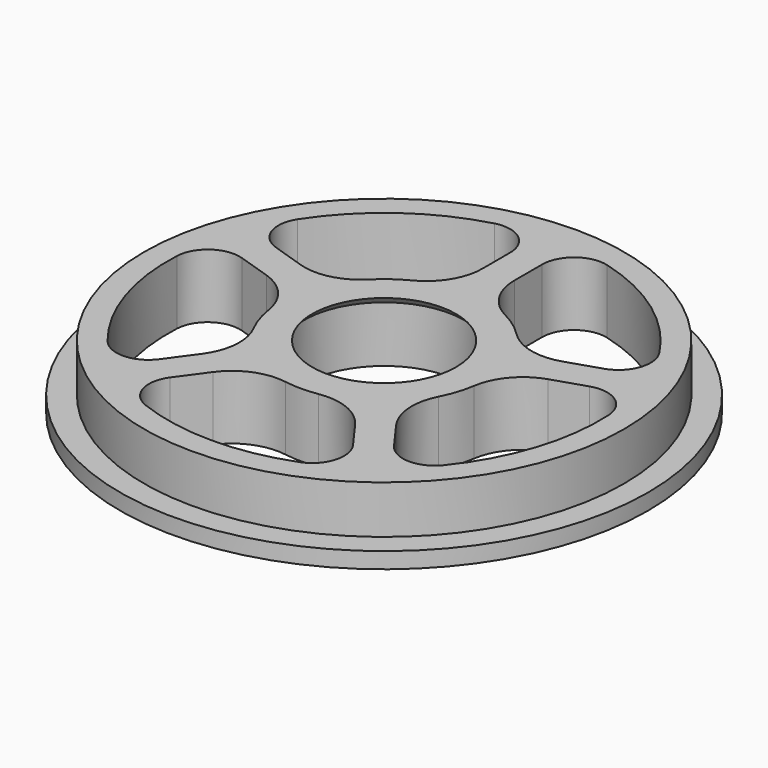
from build123d import *

# Parameters (mm, degrees)
F0_R     = 30
F0_R_2   = 10
F1_DEPTH = 8
F2_R     = 33
F2_R_2   = 30
F3_DEPTH = 2
F4_R     = 10
F4_R_2   = 9
F5_DEPTH = 1
F6_R     = 4
F7_R     = 7
F8_SIZE  = 0.99999


# Not quite as in the source:
# - a fillet or chamfer is up to 0.001 mm smaller than in the source, because OpenCascade refuses the exact size


with BuildPart() as f1:
    # F0 (on Top) → F1 (new body)
    with BuildSketch(Plane.XY):
        Circle(F0_R)
        with BuildLine():
            Line((-14.2085682852, -22.959019737), (-5.9322042833, -11.5675819574))
            ThreePointArc((-5.9322042833, -11.5675819574), (0, -13), (5.9322042833, -11.5675819574))
            Line((5.9322042833, -11.5675819574), (14.2085682852, -22.959019737))
            ThreePointArc((14.2085682852, -22.959019737), (0, -27), (-14.2085682852, -22.959019737))
        make_face(mode=Mode.SUBTRACT)
        with BuildLine():
            Line((-26.2260143945, 6.418424182), (-12.834576136, 2.0672821309))
            ThreePointArc((-12.834576136, 2.0672821309), (-12.3637347118, -4.0172209269), (-9.1682722608, -9.2164409483))
            Line((-9.1682722608, -9.2164409483), (-17.4446362627, -20.6078787278))
            ThreePointArc((-17.4446362627, -20.6078787278), (-25.67852594, -8.3434588481), (-26.2260143945, 6.418424182))
        make_face(mode=Mode.SUBTRACT)
        with BuildLine():
            Line((17.4446362627, -20.6078787278), (9.1682722608, -9.2164409483))
            ThreePointArc((9.1682722608, -9.2164409483), (12.3637347118, -4.0172209269), (12.834576136, 2.0672821309))
            Line((12.834576136, 2.0672821309), (26.2260143945, 6.418424182))
            ThreePointArc((26.2260143945, 6.418424182), (25.67852594, -8.3434588481), (17.4446362627, -20.6078787278))
        make_face(mode=Mode.SUBTRACT)
        with BuildLine():
            Line((-2, 26.9258240357), (-2, 12.8452325787))
            ThreePointArc((-2, 12.8452325787), (-7.6412082798, 10.5172209269), (-11.5985081585, 5.8715081961))
            Line((-11.5985081585, 5.8715081961), (-24.989946417, 10.2226502472))
            ThreePointArc((-24.989946417, 10.2226502472), (-15.8702018119, 21.8434588481), (-2, 26.9258240357))
        make_face(mode=Mode.SUBTRACT)
        Circle(F0_R_2, mode=Mode.SUBTRACT)
        with BuildLine():
            ThreePointArc((11.5985081585, 5.8715081961), (7.6412082798, 10.5172209269), (2, 12.8452325787))
            Line((2, 12.8452325787), (2, 26.9258240357))
            ThreePointArc((2, 26.9258240357), (15.8702018119, 21.8434588481), (24.989946417, 10.2226502472))
            Line((24.989946417, 10.2226502472), (11.5985081585, 5.8715081961))
        make_face(mode=Mode.SUBTRACT)
    extrude(amount=F1_DEPTH)

    # F2 (on face) → F3 (join)
    with BuildSketch(Plane(origin=(0, 0, 0), x_dir=(1, 0, 0), z_dir=(0, 0, -1))):
        Circle(F2_R)
        Circle(F2_R_2, mode=Mode.SUBTRACT)
    extrude(amount=-F3_DEPTH)

    # F4 (on face) → F5 (join)
    with BuildSketch(Plane.XY.offset(8)):
        Circle(F4_R)
        Circle(F4_R_2, mode=Mode.SUBTRACT)
    extrude(amount=-F5_DEPTH)

    # F6
    f6_edges = [f1.edges().sort_by_distance(p)[0] for p in [
        (-26.226014, 6.418424, 4),
        (-24.989946, 10.22265, 4),
        (-17.444636, -20.607879, 4),
        (17.444636, -20.607879, 4),
        (26.226014, 6.418424, 4),
        (-2, 26.925824, 4),
        (-14.208568, -22.95902, 4),
        (14.208568, -22.95902, 4),
        (24.989946, 10.22265, 4),
        (2, 26.925824, 4),
    ]]
    fillet(f6_edges, radius=F6_R)

    # F7
    f7_edges = [f1.edges().sort_by_distance(p)[0] for p in [
        (-12.834576, 2.067282, 4),
        (-9.168272, -9.216441, 4),
        (-5.932204, -11.567582, 4),
        (5.932204, -11.567582, 4),
        (9.168272, -9.216441, 4),
        (12.834576, 2.067282, 4),
        (11.598508, 5.871508, 4),
        (2, 12.845233, 4),
        (-2, 12.845233, 4),
        (-11.598508, 5.871508, 4),
    ]]
    fillet(f7_edges, radius=F7_R)

    # F8 (size 1 in the source; OpenCascade refuses exactly that, so slightly less here)
    f8_edges = [f1.edges().sort_by_distance(p)[0] for p in [
        (-9, 0, 7),
    ]]
    chamfer(f8_edges, length=F8_SIZE)


solid = f1.part
